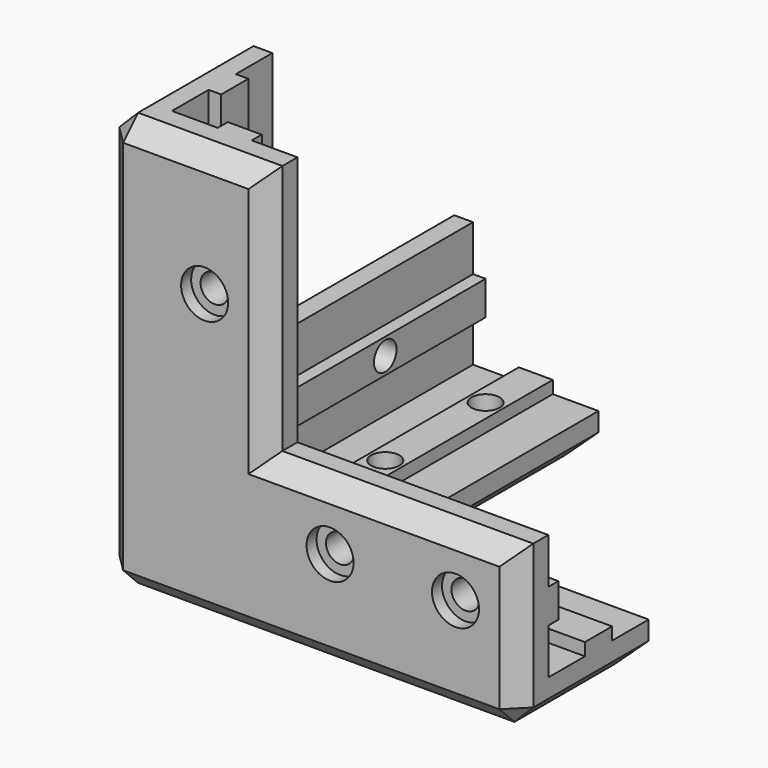
from build123d import *

# Parameters (mm, degrees)
F1_DEPTH  = 6
F3_DEPTH  = 20
F5_DEPTH  = 40
F7_DEPTH  = 60
F9_DEPTH  = 2
F11_DEPTH = 2
F13_DEPTH = 2
F14_R     = 2.25
F15_DEPTH = 8
F16_R     = 2.25
F17_DEPTH = 8
F18_R     = 3.25
F18_R_2   = 2.25
F19_DEPTH = 8.001
F20_R     = 3.75
F21_DEPTH = 2
F22_R     = 3.75
F23_DEPTH = 2
F24_R     = 3.75
F24_R_2   = 4.75
F25_DEPTH = 2
F26_SIZE  = 3


with BuildPart() as f1:
    # F0 (on Top) → F1 (new body)
    with BuildSketch(Plane.XY):
        Polygon((0, 66), (0, 0), (66, 0), (66, 26), (26, 26), (26, 66), align=None)
    extrude(amount=F1_DEPTH)

    # F2 (on face) → F3 (join)
    with BuildSketch(Plane.XY.offset(6)):
        Polygon((6, 66), (0, 66), (0, 0), (66, 0), (66, 6), (6, 6), align=None)
    extrude(amount=F3_DEPTH)

    # F4 (on face) → F5 (join)
    with BuildSketch(Plane.XY.offset(26)):
        Polygon((6, 6), (6, 26), (0, 26), (0, 0), (26, 0), (26, 6), align=None)
    extrude(amount=F5_DEPTH)

    # F6 (on face) → F7 (join)
    with BuildSketch(Plane.XY.offset(6)):
        Polygon((13.29, 6), (16, 6), (18.71, 6), (18.71, 8), (13.29, 8), align=None)
        Polygon((6, 18.71), (6, 16), (6, 13.29), (8, 13.29), (8, 18.71), align=None)
    extrude(amount=F7_DEPTH)

    # F8 (on face) → F9 (join)
    with BuildSketch(Plane.XY.offset(6)):
        Polygon((66, 13.29), (66, 16), (66, 18.71), (26, 18.71), (26, 13.29), align=None)
        Polygon((18.71, 66), (16, 66), (13.29, 66), (13.29, 26), (18.71, 26), align=None)
    extrude(amount=F9_DEPTH)

    # F10 (on face) → F11 (join)
    with BuildSketch(Plane(origin=(0, 6, 0), x_dir=(-1, 0, 0), z_dir=(0, 1, 0))):
        Polygon((-66, 18.71), (-66, 16), (-66, 13.29), (-26, 13.29), (-26, 16), (-26, 18.71), align=None)
    extrude(amount=F11_DEPTH)

    # F12 (on face) → F13 (join)
    with BuildSketch(Plane.YZ.offset(6)):
        Polygon((66, 13.29), (66, 16), (66, 18.71), (26, 18.71), (26, 13.29), align=None)
    extrude(amount=F13_DEPTH)

    # F14 (on face) → F15 (cut, through all)
    with BuildSketch(Plane.XZ):
        with Locations((56, 16)):
            Circle(F14_R)
        with Locations((16, 46)):
            Circle(F14_R)
        with Locations((36, 16)):
            Circle(F14_R)
    extrude(amount=-F15_DEPTH, mode=Mode.SUBTRACT)

    # F16 (on face) → F17 (cut, through all)
    with BuildSketch(Plane(origin=(0, 0, 0), x_dir=(0, -1, 0), z_dir=(-1, 0, 0))):
        with Locations((-16, 56)):
            Circle(F16_R)
        with Locations((-46, 16)):
            Circle(F16_R)
        with Locations((-16, 36)):
            Circle(F16_R)
    extrude(amount=-F17_DEPTH, mode=Mode.SUBTRACT)

    # F18 (on face) → F19 (cut, through all)
    with BuildSketch(Plane(origin=(0, 0, 0), x_dir=(1, 0, 0), z_dir=(0, 0, -1))):
        with Locations((16, -16)):
            Circle(F18_R)
        with Locations((46, -16)):
            Circle(F18_R_2)
        with Locations((16, -56)):
            Circle(F18_R_2)
        with Locations((16, -36)):
            Circle(F18_R_2)
    extrude(amount=-F19_DEPTH, mode=Mode.SUBTRACT)

    # F20 (on face) → F21 (cut)
    with BuildSketch(Plane.XZ):
        with Locations((16, 46)):
            Circle(F20_R)
        with Locations((36, 16)):
            Circle(F20_R)
        with Locations((56, 16)):
            Circle(F20_R)
    extrude(amount=-F21_DEPTH, mode=Mode.SUBTRACT)

    # F22 (on face) → F23 (cut)
    with BuildSketch(Plane(origin=(0, 0, 0), x_dir=(0, -1, 0), z_dir=(-1, 0, 0))):
        with Locations((-16, 56)):
            Circle(F22_R)
        with Locations((-46, 16)):
            Circle(F22_R)
        with Locations((-16, 36)):
            Circle(F22_R)
    extrude(amount=-F23_DEPTH, mode=Mode.SUBTRACT)

    # F24 (on face) → F25 (cut)
    with BuildSketch(Plane(origin=(0, 0, 0), x_dir=(1, 0, 0), z_dir=(0, 0, -1))):
        with Locations((16, -56)):
            Circle(F24_R)
        with Locations((16, -16)):
            Circle(F24_R_2)
        with Locations((46, -16)):
            Circle(F24_R)
        with Locations((16, -36)):
            Circle(F24_R)
    extrude(amount=-F25_DEPTH, mode=Mode.SUBTRACT)

    # F26
    f26_edges = [f1.edges().sort_by_distance(p)[0] for p in [
        (33, 0, 0),
        (0, 33, 0),
        (0, 0, 33),
        (0, 26, 46),
        (0, 46, 26),
        (26, 0, 46),
        (46, 0, 26),
        (0, 13, 66),
        (13, 0, 66),
        (0, 66, 13),
        (13, 66, 0),
        (66, 0, 13),
        (66, 13, 0),
        (46, 26, 0),
        (26, 46, 0),
    ]]
    chamfer(f26_edges, length=F26_SIZE)


solid = f1.part
